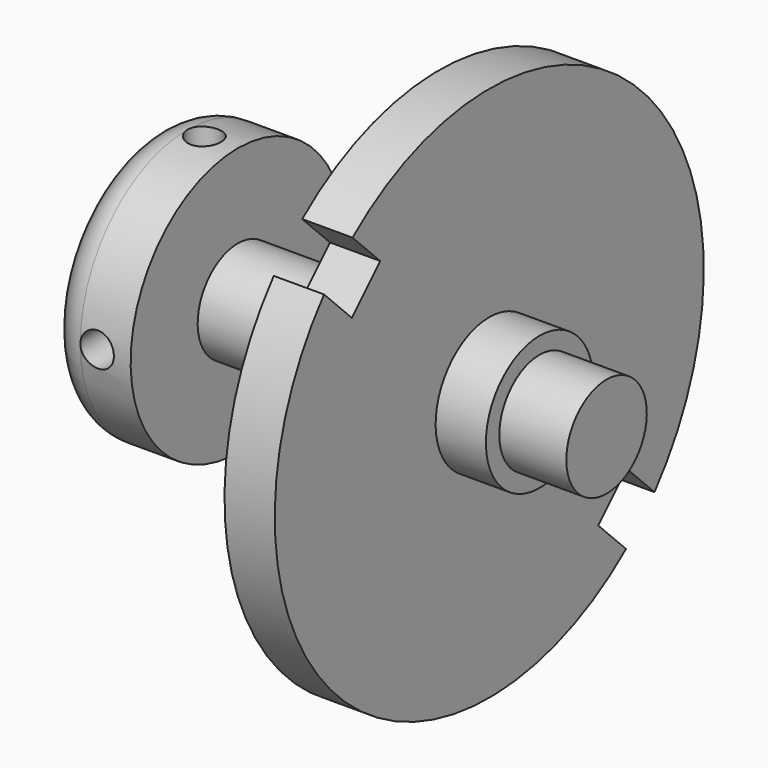
from build123d import *

# Parameters (mm, degrees)
F3_R            = 6.35
F4_DEPTH        = 16.002
F4_COPIES_COUNT = 4
F6_DEPTH        = 25.4
F7_R            = 9.525
F8_DEPTH        = 20.828
F9_SIZE         = 1.524


# Not quite as in the source:
# - a pattern or mirror of a feature is missing from the dataset's text; its kind, count and spacing are read off the source's solid


with BuildPart() as f1:
    # F0 (on Front) → F1 (revolve)
    with BuildSketch(Plane.XZ):
        with BuildLine():
            Line((0, 38.1), (0, 0))
            Line((0, 0), (171.45, 0))
            Line((171.45, 0), (171.45, 19.05))
            Line((171.45, 19.05), (146.05, 19.05))
            Line((146.05, 19.05), (146.05, 25.4))
            Line((146.05, 25.4), (127, 25.4))
            Line((127, 25.4), (127, 101.6))
            Line((127, 101.6), (107.95, 101.6))
            Line((107.95, 101.6), (107.95, 19.05))
            Line((107.95, 19.05), (31.75, 19.05))
            Line((31.75, 19.05), (31.75, 50.8))
            Line((31.75, 50.8), (12.7, 50.8))
            ThreePointArc((12.7, 50.8), (3.7197438789, 47.0802561211), (0, 38.1))
        make_face()
    revolve(axis=Axis((85.725, 0, 0), (1, 0, 0)))

    # F3 (on offset) → F4 (cut)
    with BuildSketch(Plane.XZ.offset(50.8)):
        with Locations((19.05, 0)):
            Circle(F3_R)
    f4 = extrude(amount=-F4_DEPTH, mode=Mode.SUBTRACT)

    # F4_copies: F4 ×4 about axis
    f4_copies_axis = Axis((0, 0, 0), (1, 0, 0))
    for i in range(1, F4_COPIES_COUNT):
        add(f4.rotate(f4_copies_axis, i * 360 / F4_COPIES_COUNT), mode=Mode.SUBTRACT)

    # F5 (on face) → F6 (cut)
    with BuildSketch(Plane(origin=(107.95, 0, 0), x_dir=(0, -1, 0), z_dir=(-1, 0, 0))):
        with BuildLine():
            ThreePointArc((-64.7904479797, -78.2608321613), (-71.8420489686, -71.8420489686), (-78.2608321613, -64.7904479797))
            Line((-78.2608321613, -64.7904479797), (-92.047625241, -78.5772410594))
            Line((-92.047625241, -78.5772410594), (-78.5772410594, -92.047625241))
            Line((-78.5772410594, -92.047625241), (-64.7904479797, -78.2608321613))
        make_face()
        with BuildLine():
            Line((-65.1068568778, -51.6364726961), (-78.2608321613, -64.7904479797))
            ThreePointArc((-78.2608321613, -64.7904479797), (-71.8420489686, -71.8420489686), (-64.7904479797, -78.2608321613))
            Line((-64.7904479797, -78.2608321613), (-51.6364726961, -65.1068568778))
            Line((-51.6364726961, -65.1068568778), (-65.1068568778, -51.6364726961))
        make_face()
        with BuildLine():
            ThreePointArc((78.2608321613, 64.7904479797), (71.8420489686, 71.8420489686), (64.7904479797, 78.2608321613))
            Line((64.7904479797, 78.2608321613), (51.6364726961, 65.1068568778))
            Line((51.6364726961, 65.1068568778), (65.1068568778, 51.6364726961))
            Line((65.1068568778, 51.6364726961), (78.2608321613, 64.7904479797))
        make_face()
        with BuildLine():
            Line((92.047625241, 78.5772410594), (78.5772410594, 92.047625241))
            Line((78.5772410594, 92.047625241), (64.7904479797, 78.2608321613))
            ThreePointArc((64.7904479797, 78.2608321613), (71.8420489686, 71.8420489686), (78.2608321613, 64.7904479797))
            Line((78.2608321613, 64.7904479797), (92.047625241, 78.5772410594))
        make_face()
    extrude(amount=-F6_DEPTH, mode=Mode.SUBTRACT)

    # F7 (on face) → F8 (join)
    with BuildSketch(Plane(origin=(107.95, 0, 0), x_dir=(0, -1, 0), z_dir=(-1, 0, 0))):
        with Locations((53.8815367264, -53.8815367264)):
            Circle(F7_R)
        with Locations((-53.8815367264, 53.8815367264)):
            Circle(F7_R)
    extrude(amount=F8_DEPTH)

    # F9
    f9_edges = [f1.edges().sort_by_distance(p)[0] for p in [
        (87.122, 63.406537, 53.881537),
        (87.122, -44.356537, -53.881537),
    ]]
    chamfer(f9_edges, length=F9_SIZE)


solid = f1.part
